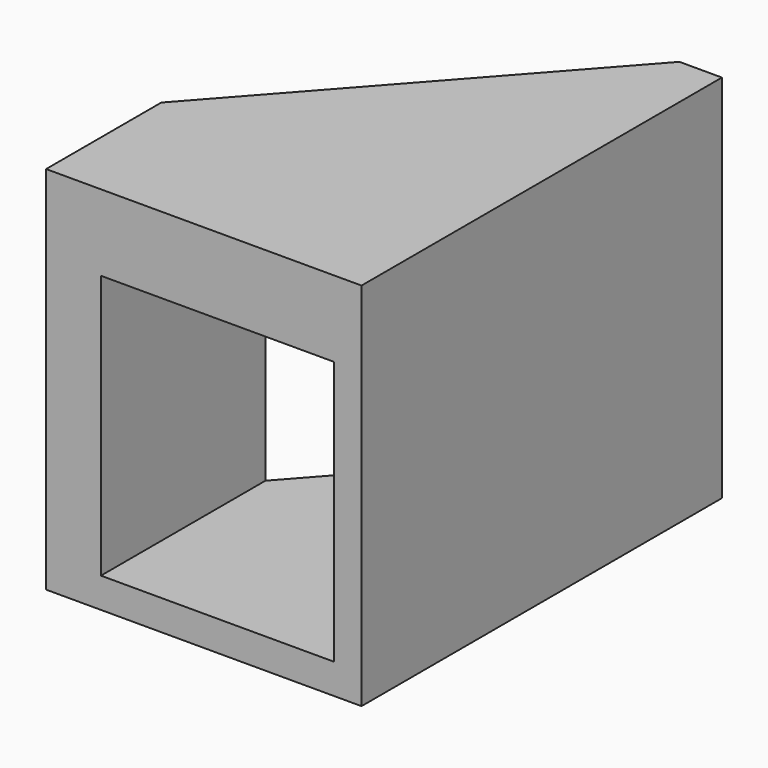
from build123d import *

# Parameters (mm, degrees)
F0_W     = 23
F0_H     = 27
F1_DEPTH = 32.85
F2_W     = 17
F2_H     = 19.25
F3_DEPTH = 32.851
F5_DEPTH = 27.001
F7_D     = 3.25
F7_DEPTH = 8
F7_TIP   = 0.9763985059


# Not quite as in the source:
# - a feature names something its author has since deleted; it is built from what else it names


with BuildPart() as f1:
    # F0 (on Front) → F1 (new body)
    with BuildSketch(Plane.XZ):
        Rectangle(F0_W, F0_H)
    extrude(amount=F1_DEPTH)

    # F2 (on face) → F3 (cut, through all)
    with BuildSketch(Plane.XZ.offset(32.85)):
        with Locations((1, -1.675)):
            Rectangle(F2_W, F2_H)
    extrude(amount=-F3_DEPTH, mode=Mode.SUBTRACT)

    # F4 (on face) → F5 (cut, through all)
    with BuildSketch(Plane.XY.offset(13.5)):
        Polygon((-11.5, -22.35), (8.4, 0), (-11.5, 0), align=None)
    extrude(amount=-F5_DEPTH, mode=Mode.SUBTRACT)

    # F7
    with Locations(Plane(origin=(-11.5, 0, 0), x_dir=(0, -1, 0), z_dir=(-1, 0, 0))):
        with Locations((25.7, 7.4)):
            Hole(F7_D / 2, depth=F7_DEPTH)
            with Locations((0, 0, -(F7_DEPTH + F7_TIP / 2))):  # 118° drill point
                Cone(0, F7_D / 2, F7_TIP, mode=Mode.SUBTRACT)


solid = f1.part
